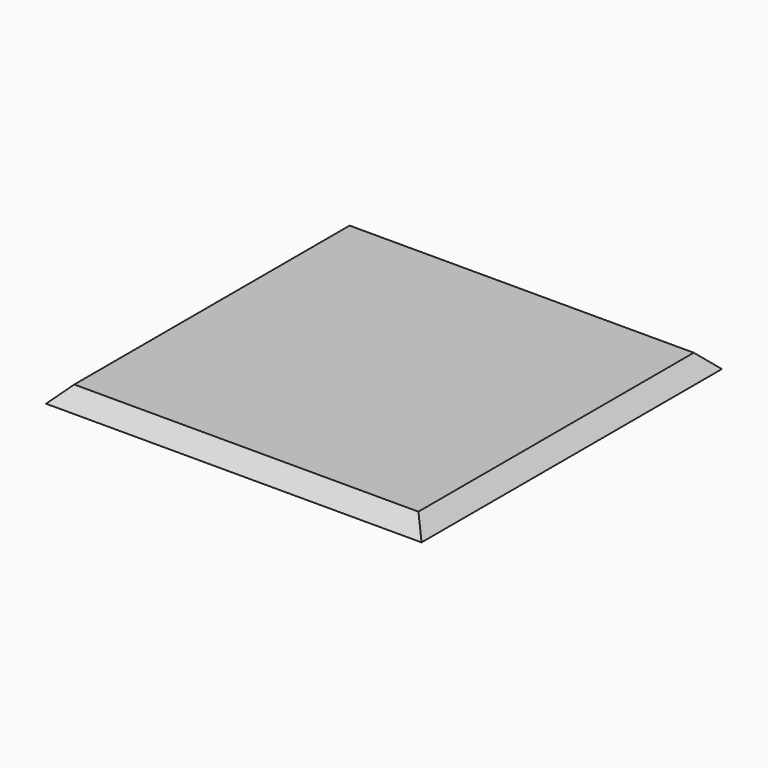
from build123d import *

# Parameters (mm, degrees)
F0_W     = 76.2
F0_H     = 76.2
F1_DEPTH = 3.175
F2_SIZE  = 3.17499


# Not quite as in the source:
# - a fillet or chamfer is up to 0.001 mm smaller than in the source, because OpenCascade refuses the exact size


with BuildPart() as f1:
    # F0 (on Top) → F1 (new body)
    with BuildSketch(Plane.XY):
        with Locations((38.1, 38.1)):
            Rectangle(F0_W, F0_H)
    extrude(amount=F1_DEPTH)

    # F2 (size 3.175 in the source; OpenCascade refuses exactly that, so slightly less here)
    f2_edges = [f1.edges().sort_by_distance(p)[0] for p in [
        (38.1, 76.2, 3.175),
        (76.2, 38.1, 3.175),
        (38.1, 0, 3.175),
        (0, 38.1, 3.175),
    ]]
    chamfer(f2_edges, length=F2_SIZE)


solid = f1.part
